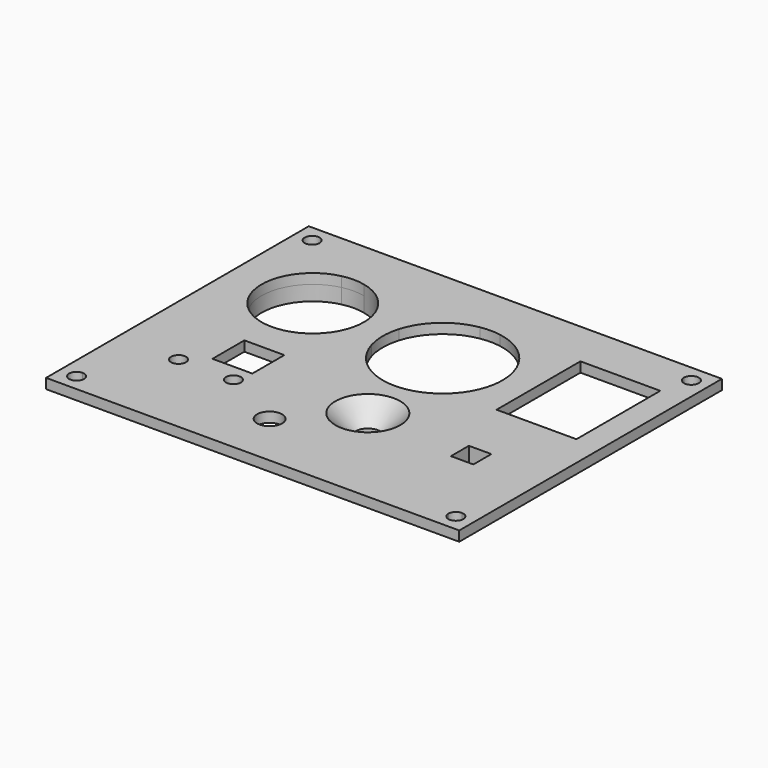
from build123d import *

# Parameters (mm, degrees)
F0_W     = 82.8
F0_H     = 65.8
F0_R     = 2.5
F0_W_2   = 8
F0_H_2   = 8
F0_R_2   = 5.5
F0_W_3   = 6.5
F0_H_3   = 6.5
F0_W_4   = 4.5
F0_H_4   = 4.5
F0_R_3   = 1.5
F1_DEPTH = 2
F2_DEPTH = 3
F3_SIZE  = 4


# Not quite as in the source:
# - a feature names something its author has since deleted; it is built from what else it names


with BuildPart() as f1:
    # F0 (on Top) → F1 (new body)
    with BuildSketch(Plane.XY):
        with Locations((0.3088639305, 12.5479439557)):
            Rectangle(F0_W, F0_H)
        with BuildLine():
            ThreePointArc((-37.6911360695, 40.5479439557), (-38.7517962413, 43.1086041274), (-36.1911360695, 42.0479439557))
            Line((-36.1911360695, 42.0479439557), (36.8088639305, 42.0479439557))
            ThreePointArc((36.8088639305, 42.0479439557), (38.3088639305, 43.5479439557), (39.8088639305, 42.0479439557))
            ThreePointArc((39.8088639305, 42.0479439557), (39.3695241023, 40.9872837839), (38.3088639305, 40.5479439557))
            Line((38.3088639305, 40.5479439557), (38.3088639305, -15.4520560443))
            ThreePointArc((38.3088639305, -15.4520560443), (39.3695241023, -15.8913958726), (39.8088639305, -16.9520560443))
            ThreePointArc((39.8088639305, -16.9520560443), (38.3088639305, -18.4520560443), (36.8088639305, -16.9520560443))
            Line((36.8088639305, -16.9520560443), (-36.1911360695, -16.9520560443))
            ThreePointArc((-36.1911360695, -16.9520560443), (-38.7517962413, -18.0127162161), (-37.6911360695, -15.4520560443))
            Line((-37.6911360695, -15.4520560443), (-37.6911360695, 40.5479439557))
        make_face(mode=Mode.SUBTRACT)
        with BuildLine():
            Line((36.8088639305, 42.0479439557), (-36.1911360695, 42.0479439557))
            ThreePointArc((-36.1911360695, 42.0479439557), (-36.6304758977, 40.9872837839), (-37.6911360695, 40.5479439557))
            Line((-37.6911360695, 40.5479439557), (-37.6911360695, -15.4520560443))
            ThreePointArc((-37.6911360695, -15.4520560443), (-36.6304758977, -15.8913958726), (-36.1911360695, -16.9520560443))
            Line((-36.1911360695, -16.9520560443), (36.8088639305, -16.9520560443))
            ThreePointArc((36.8088639305, -16.9520560443), (37.2482037587, -15.8913958726), (38.3088639305, -15.4520560443))
            Line((38.3088639305, -15.4520560443), (38.3088639305, 40.5479439557))
            ThreePointArc((38.3088639305, 40.5479439557), (37.2482037587, 40.9872837839), (36.8088639305, 42.0479439557))
        make_face()
        with BuildLine():
            Line((-35.2911360695, 27.8064392387), (-35.2911360695, 35.4479439557))
            Line((-35.2911360695, 35.4479439557), (-29.4450181015, 35.4479439557))
            ThreePointArc((-29.4450181015, 35.4479439557), (-24.2911360695, 36.6979439557), (-19.1372540375, 35.4479439557))
            Line((-19.1372540375, 35.4479439557), (-8.2911360695, 35.4479439557))
            Line((-8.2911360695, 35.4479439557), (1.2206639384, 35.4479439557))
            ThreePointArc((1.2206639384, 35.4479439557), (3.2088639305, 35.6137958751), (5.1970639225, 35.4479439557))
            Line((5.1970639225, 35.4479439557), (14.7088639305, 35.4479439557))
            Line((14.7088639305, 35.4479439557), (20.7088639305, 35.4479439557))
            Line((20.7088639305, 35.4479439557), (20.7088639305, 36.2488545371))
            Line((20.7088639305, 36.2488545371), (36.7088639305, 36.2488545371))
            Line((36.7088639305, 36.2488545371), (36.7088639305, 15.2488545371))
            Line((36.7088639305, 15.2488545371), (34.7088639305, 15.2488545371))
            Line((34.7088639305, 15.2488545371), (34.7088639305, -14.2511454629))
            Line((34.7088639305, -14.2511454629), (-35.2911360695, -14.5520560443))
            Line((-35.2911360695, -14.5520560443), (-35.2911360695, 23.0894486726))
            ThreePointArc((-35.2911360695, 23.0894486726), (-35.5411360695, 25.4479439557), (-35.2911360695, 27.8064392387))
        make_face(mode=Mode.SUBTRACT)
        with BuildLine():
            Line((-8.2911360695, 35.4479439557), (-19.1372540375, 35.4479439557))
            ThreePointArc((-19.1372540375, 35.4479439557), (-14.6853130215, 31.3037670037), (-13.0411360695, 25.4479439557))
            ThreePointArc((-13.0411360695, 25.4479439557), (-23.105281947, 14.260618538), (-35.2911360695, 23.0894486726))
            Line((-35.2911360695, 23.0894486726), (-35.2911360695, -14.5520560443))
            Line((-35.2911360695, -14.5520560443), (34.7088639305, -14.2511454629))
            Line((34.7088639305, -14.2511454629), (34.7088639305, 15.2488545371))
            Line((34.7088639305, 15.2488545371), (20.7088639305, 15.2488545371))
            Line((20.7088639305, 15.2488545371), (20.7088639305, 35.4479439557))
            Line((20.7088639305, 35.4479439557), (14.7088639305, 35.4479439557))
            Line((14.7088639305, 35.4479439557), (14.7088639305, 27.0416231753))
            ThreePointArc((14.7088639305, 27.0416231753), (15.0832060175, 25.3458466827), (15.2088639305, 23.6137958751))
            ThreePointArc((15.2088639305, 23.6137958751), (15.0832060175, 21.8817450676), (14.7088639305, 20.1859685749))
            Line((14.7088639305, 20.1859685749), (14.7088639305, 12.4479439557))
            Line((14.7088639305, 12.4479439557), (7.604742786, 12.4479439557))
            ThreePointArc((7.604742786, 12.4479439557), (3.2088639305, 11.6137958751), (-1.187014925, 12.4479439557))
            Line((-1.187014925, 12.4479439557), (-8.2911360695, 12.4479439557))
            Line((-8.2911360695, 12.4479439557), (-8.2911360695, 20.1859685749))
            ThreePointArc((-8.2911360695, 20.1859685749), (-8.7911360695, 23.6137958751), (-8.2911360695, 27.0416231753))
            Line((-8.2911360695, 27.0416231753), (-8.2911360695, 35.4479439557))
        make_face()
        with Locations((-5.0911360695, -9.3520560443)):
            Circle(F0_R, mode=Mode.SUBTRACT)
        with Locations((-28.7911360695, -2.5520560443)):
            Circle(F0_R, mode=Mode.SUBTRACT)
        with Locations((-20.7911360695, 4.9479439557)):
            Rectangle(F0_W_2, F0_H_2, mode=Mode.SUBTRACT)
        with Locations((-17.7911360695, -2.5520560443)):
            Circle(F0_R, mode=Mode.SUBTRACT)
        with Locations((5.7088639305, 1.7488545371)):
            Circle(F0_R_2, mode=Mode.SUBTRACT)
        with Locations((27.2088639305, 0.7488545371)):
            Rectangle(F0_W_3, F0_H_3, mode=Mode.SUBTRACT)
        with Locations((5.7088639305, 1.7488545371)):
            Circle(F0_R_2)
        with Locations((5.7088639305, 1.7488545371)):
            Circle(F0_R, mode=Mode.SUBTRACT)
        with BuildLine():
            Line((-26.5411360695, 35.4479439557), (-29.4450181015, 35.4479439557))
            ThreePointArc((-29.4450181015, 35.4479439557), (-33.2261864197, 32.2836864346), (-35.2911360695, 27.8064392387))
            Line((-35.2911360695, 27.8064392387), (-35.2911360695, 23.0894486726))
            ThreePointArc((-35.2911360695, 23.0894486726), (-23.105281947, 14.260618538), (-13.0411360695, 25.4479439557))
            ThreePointArc((-13.0411360695, 25.4479439557), (-14.6853130215, 31.3037670037), (-19.1372540375, 35.4479439557))
            Line((-19.1372540375, 35.4479439557), (-22.0411360695, 35.4479439557))
            ThreePointArc((-22.0411360695, 35.4479439557), (-16.2872307727, 31.8510681931), (-14.0411360695, 25.4479439557))
            ThreePointArc((-14.0411360695, 25.4479439557), (-30.694260307, 17.4440386589), (-26.5411360695, 35.4479439557))
        make_face()
        with Locations((27.2088639305, 0.7488545371)):
            Rectangle(F0_W_3, F0_H_3)
        with Locations((27.2088639305, 0.7488545371)):
            Rectangle(F0_W_4, F0_H_4, mode=Mode.SUBTRACT)
        with BuildLine():
            Line((1.2206639384, 35.4479439557), (-8.2911360695, 35.4479439557))
            Line((-8.2911360695, 35.4479439557), (-8.2911360695, 27.0416231753))
            ThreePointArc((-8.2911360695, 27.0416231753), (-4.7377983891, 32.6054897077), (1.2206639384, 35.4479439557))
        make_face()
        with BuildLine():
            Line((14.7088639305, 35.4479439557), (5.1970639225, 35.4479439557))
            ThreePointArc((5.1970639225, 35.4479439557), (11.1555262501, 32.6054897077), (14.7088639305, 27.0416231753))
            Line((14.7088639305, 27.0416231753), (14.7088639305, 35.4479439557))
        make_face()
        with Locations((-17.7911360695, -2.5520560443)):
            Circle(F0_R)
        with Locations((-17.7911360695, -2.5520560443)):
            Circle(F0_R_3, mode=Mode.SUBTRACT)
        with Locations((-28.7911360695, -2.5520560443)):
            Circle(F0_R)
        with Locations((-28.7911360695, -2.5520560443)):
            Circle(F0_R_3, mode=Mode.SUBTRACT)
        with BuildLine():
            ThreePointArc((-1.187014925, 12.4479439557), (-5.6307626114, 15.4983166779), (-8.2911360695, 20.1859685749))
            Line((-8.2911360695, 20.1859685749), (-8.2911360695, 12.4479439557))
            Line((-8.2911360695, 12.4479439557), (-1.187014925, 12.4479439557))
        make_face()
        with BuildLine():
            Line((14.7088639305, 12.4479439557), (14.7088639305, 20.1859685749))
            ThreePointArc((14.7088639305, 20.1859685749), (12.0484904723, 15.4983166779), (7.604742786, 12.4479439557))
            Line((7.604742786, 12.4479439557), (14.7088639305, 12.4479439557))
        make_face()
        with BuildLine():
            Line((-29.4450181015, 35.4479439557), (-35.2911360695, 35.4479439557))
            Line((-35.2911360695, 35.4479439557), (-35.2911360695, 27.8064392387))
            ThreePointArc((-35.2911360695, 27.8064392387), (-33.2261864197, 32.2836864346), (-29.4450181015, 35.4479439557))
        make_face()
        with BuildLine():
            ThreePointArc((-19.1372540375, 35.4479439557), (-24.2911360695, 36.6979439557), (-29.4450181015, 35.4479439557))
            Line((-29.4450181015, 35.4479439557), (-26.5411360695, 35.4479439557))
            ThreePointArc((-26.5411360695, 35.4479439557), (-24.2911360695, 35.6979439557), (-22.0411360695, 35.4479439557))
            Line((-22.0411360695, 35.4479439557), (-19.1372540375, 35.4479439557))
        make_face()
        with BuildLine():
            Line((-35.2911360695, 23.0894486726), (-35.2911360695, 27.8064392387))
            ThreePointArc((-35.2911360695, 27.8064392387), (-35.5411360695, 25.4479439557), (-35.2911360695, 23.0894486726))
        make_face()
    extrude(amount=F1_DEPTH)

    # F0 (on Top) → F2 (join)
    with BuildSketch(Plane.XY):
        with Locations((27.2088639305, 0.7488545371)):
            Rectangle(F0_W_3, F0_H_3)
        with Locations((27.2088639305, 0.7488545371)):
            Rectangle(F0_W_4, F0_H_4, mode=Mode.SUBTRACT)
        with BuildLine():
            Line((-26.5411360695, 35.4479439557), (-29.4450181015, 35.4479439557))
            ThreePointArc((-29.4450181015, 35.4479439557), (-33.2261864197, 32.2836864346), (-35.2911360695, 27.8064392387))
            Line((-35.2911360695, 27.8064392387), (-35.2911360695, 23.0894486726))
            ThreePointArc((-35.2911360695, 23.0894486726), (-23.105281947, 14.260618538), (-13.0411360695, 25.4479439557))
            ThreePointArc((-13.0411360695, 25.4479439557), (-14.6853130215, 31.3037670037), (-19.1372540375, 35.4479439557))
            Line((-19.1372540375, 35.4479439557), (-22.0411360695, 35.4479439557))
            ThreePointArc((-22.0411360695, 35.4479439557), (-16.2872307727, 31.8510681931), (-14.0411360695, 25.4479439557))
            ThreePointArc((-14.0411360695, 25.4479439557), (-30.694260307, 17.4440386589), (-26.5411360695, 35.4479439557))
        make_face()
        with Locations((-17.7911360695, -2.5520560443)):
            Circle(F0_R)
        with Locations((-17.7911360695, -2.5520560443)):
            Circle(F0_R_3, mode=Mode.SUBTRACT)
        with Locations((5.7088639305, 1.7488545371)):
            Circle(F0_R_2)
        with Locations((5.7088639305, 1.7488545371)):
            Circle(F0_R, mode=Mode.SUBTRACT)
        with BuildLine():
            ThreePointArc((-19.1372540375, 35.4479439557), (-24.2911360695, 36.6979439557), (-29.4450181015, 35.4479439557))
            Line((-29.4450181015, 35.4479439557), (-26.5411360695, 35.4479439557))
            ThreePointArc((-26.5411360695, 35.4479439557), (-24.2911360695, 35.6979439557), (-22.0411360695, 35.4479439557))
            Line((-22.0411360695, 35.4479439557), (-19.1372540375, 35.4479439557))
        make_face()
        with Locations((-28.7911360695, -2.5520560443)):
            Circle(F0_R)
        with Locations((-28.7911360695, -2.5520560443)):
            Circle(F0_R_3, mode=Mode.SUBTRACT)
        with BuildLine():
            Line((-35.2911360695, 23.0894486726), (-35.2911360695, 27.8064392387))
            ThreePointArc((-35.2911360695, 27.8064392387), (-35.5411360695, 25.4479439557), (-35.2911360695, 23.0894486726))
        make_face()
    extrude(amount=-F2_DEPTH)

    # F3
    f3_edges = [f1.edges().sort_by_distance(p)[0] for p in [
        (3.208864, 1.748855, 2),
    ]]
    chamfer(f3_edges, length=F3_SIZE)


solid = f1.part
